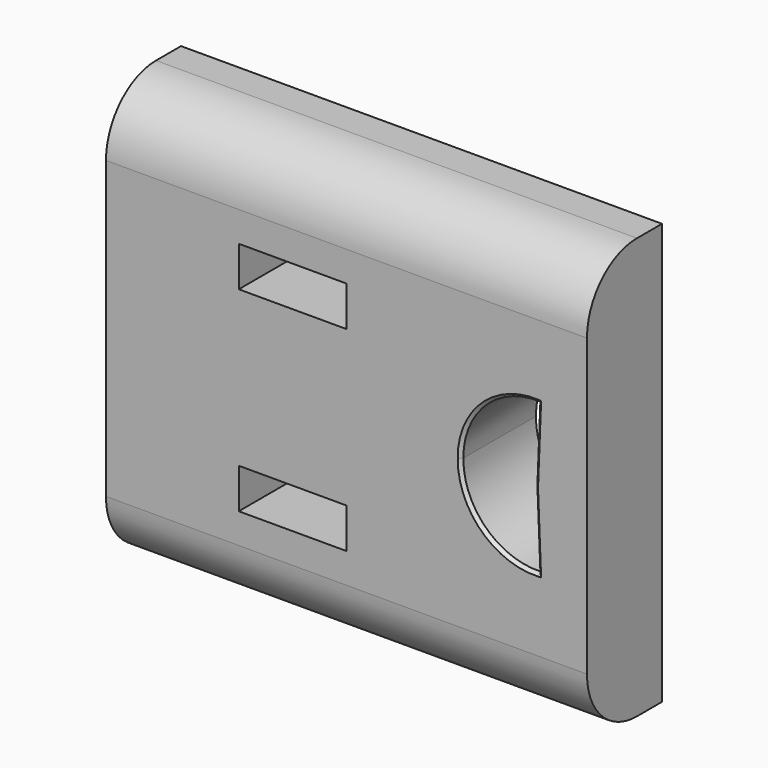
from build123d import *

# Parameters (mm, degrees)
F0_W         = 39.0713959932
F0_H         = 34.1874808073
F0_W_2       = 8.7503567338
F0_H_2       = 3.2559484243
F1_DEPTH     = 7.62
F2_R         = 5.08
F3_R         = 5.08
F4_T2_ANGLE  = 99.0884829953
F4_T4_ANGLE  = 99.0884829953
F4_T8_DEPTH  = 7.3218336241
F4_S9_R      = 6.0154186662
F4_T10_DEPTH = 5
F4_T14_DEPTH = 7.3218336241
F4_S15_R     = 6.0154186662
F4_T16_DEPTH = 5
F4_T21_DEPTH = 7.3218336241
F4_S22_R     = 6.0154186662
F4_T23_DEPTH = 5
F4_T26_ANGLE = 105.3128275547
F4_T33_ANGLE = 105.3128275547
F4_T37_DEPTH = 7.3218336241
F4_S38_R     = 6.0154186662
F4_T39_DEPTH = 5


# Not quite as in the source:
# - a fillet or chamfer that OpenCascade refuses, or shapes differently, is made with other operations: its cross-section is extruded or revolved along the edge and cut away or added


with BuildPart() as f1:
    # F0 (on Front) → F1 (new body)
    with BuildSketch(Plane.XZ):
        with Locations((19.5356979966, 17.0937404037)):
            Rectangle(F0_W, F0_H)
        with Locations((15.1605196297, 9.1573596001)):
            Rectangle(F0_W_2, F0_H_2, mode=Mode.SUBTRACT)
        with Locations((15.1605196297, 25.0301212072)):
            Rectangle(F0_W_2, F0_H_2, mode=Mode.SUBTRACT)
        with BuildLine():
            ThreePointArc((28.8283239088, 17.0937404037), (30.6523842077, 21.4714728973), (35.0814722478, 23.1670308858))
            Line((35.0814722478, 23.1670308858), (34.8434170056, 17.1563244854))
            Line((34.8434170056, 17.1563244854), (34.8434170056, 17.0311563219))
            Line((34.8434170056, 17.0311563219), (35.0814722478, 11.0204499215))
            ThreePointArc((35.0814722478, 11.0204499215), (30.6523842077, 12.71600791), (28.8283239088, 17.0937404037))
        make_face(mode=Mode.SUBTRACT)
    extrude(amount=F1_DEPTH)

    # F2
    f2_edges = [f1.edges().sort_by_distance(p)[0] for p in [
        (19.535698, -7.62, 34.187481),
    ]]
    fillet(f2_edges, radius=F2_R)

    # F3
    f3_edges = [f1.edges().sort_by_distance(p)[0] for p in [
        (19.535698, -7.62, 0),
    ]]
    fillet(f3_edges, radius=F3_R)

    # F4: chamfer of 0.254 on 4 edges, made by hand

    # F4_s1 → F4_t2 (revolve, cut)
    with BuildSketch(Plane(origin=(35.4623142005, 0, 1.4044921235), x_dir=(0, 1, 0), z_dir=(0.9992166354, 0, 0.0395741769))):
        Polygon((-7.62, 9.3694965041), (-7.366, 9.6234965041), (-7.62, 9.6234965041), align=None)
    revolve(axis=Axis((34.8434170056, -7.62, 17.0311563219), (0, 1, 0)), revolution_arc=F4_T2_ANGLE, mode=Mode.SUBTRACT)

    # F4_s3 → F4_t4 (revolve, cut)
    with BuildSketch(Plane(origin=(-1.5316236266, 0, 12.8056905764), x_dir=(0, 1, 0), z_dir=(0.1187584985, 0, -0.9929231688))):
        Polygon((-7.62, 30.3648766921), (-7.366, 30.6188766921), (-7.62, 30.6188766921), align=None)
    revolve(axis=Axis((34.8434170056, -7.62, 17.1563244854), (0, 1, 0)), revolution_arc=F4_T4_ANGLE, mode=Mode.SUBTRACT)


with BuildPart() as f4_tool6:
    # F4_s7 → F4_t8 (new body)
    with BuildSketch(Plane(origin=(0.9968897612, 0, 25.170677246), x_dir=(0, 1, 0), z_dir=(-0.0395741769, 0, -0.9992166354))):
        Polygon((-7.62, 34.3911744878), (-7.366, 34.1371744878), (-7.62, 34.1371744878), align=None)
    extrude(amount=F4_T8_DEPTH)

    # F4_s9 → F4_t10 (intersect, symmetric)
    with BuildSketch(Plane.XZ.offset(7.5)):
        with Locations((34.8434170056, 17.1563244854)):
            Circle(F4_S9_R)
    extrude(amount=F4_T10_DEPTH, both=True, mode=Mode.INTERSECT)


with BuildPart() as f1_1:
    add(f1.part)

    # F4_t5: cut F4_tool6
    add(f4_tool6.part, mode=Mode.SUBTRACT)


with BuildPart() as f4_tool12:
    # F4_s13 → F4_t14 (new body)
    with BuildSketch(Plane(origin=(-0.6447473432, 0, 16.2793599777), x_dir=(0, 1, 0), z_dir=(0.0395741769, 0, -0.9992166354))):
        Polygon((-7.62, 35.7441158998), (-7.366, 35.4901158998), (-7.62, 35.4901158998), align=None)
    extrude(amount=F4_T14_DEPTH)

    # F4_s15 → F4_t16 (intersect, symmetric)
    with BuildSketch(Plane.XZ.offset(7.5)):
        with Locations((34.8434170056, 17.0311563219)):
            Circle(F4_S15_R)
    extrude(amount=F4_T16_DEPTH, both=True, mode=Mode.INTERSECT)


with BuildPart() as f1_2:
    add(f1_1.part)

    # F4_t11: cut F4_tool12
    add(f4_tool12.part, mode=Mode.SUBTRACT)


with BuildPart() as f4_tool19:
    # F4_s20 → F4_t21 (new body)
    with BuildSketch(Plane(origin=(-0.6447473432, 0, 16.2793599777), x_dir=(0, 1, 0), z_dir=(0.0395741769, 0, -0.9992166354))):
        Polygon((-7.62, 35.7441158998), (-7.366, 35.4901158998), (-7.62, 35.4901158998), align=None)
    extrude(amount=F4_T21_DEPTH)

    # F4_s22 → F4_t23 (cut, symmetric)
    with BuildSketch(Plane.XZ.offset(7.5)):
        with Locations((34.8434170056, 17.0311563219)):
            Circle(F4_S22_R)
    extrude(amount=F4_T23_DEPTH, both=True, mode=Mode.SUBTRACT)


with BuildPart() as f4_tool24:
    # F4_s25 → F4_t26 (revolve)
    with BuildSketch(Plane(origin=(36.5710723448, 0, 5.4606046716), x_dir=(0, 1, 0), z_dir=(0.9890355378, 0, 0.1476777062))):
        Polygon((-7.62, 5.4294042858), (-7.366, 5.6834042858), (-7.62, 5.6834042858), align=None)
    revolve(axis=Axis((34.8434170056, -7.62, 17.0311563219), (0, 1, 0)), revolution_arc=F4_T26_ANGLE)

    split(bisect_by=Plane(origin=(35.4623142005, 0, 1.4044921235), x_dir=(0, 1, 0), z_dir=(0.9992166354, 0, 0.0395741769)), keep=Keep.TOP)


with BuildPart() as f4_tool19_1:
    add(f4_tool19.part)

    # F4_t28: intersect F4_tool24
    add(f4_tool24.part, mode=Mode.INTERSECT)


with BuildPart() as f1_3:
    add(f1_2.part)

    # F4_t17: cut F4_tool19
    add(f4_tool19_1.part, mode=Mode.SUBTRACT)


with BuildPart() as f4_tool31:
    # F4_s32 → F4_t33 (revolve)
    with BuildSketch(Plane(origin=(-1.5316236266, 0, 12.8056905764), x_dir=(0, 1, 0), z_dir=(0.1187584985, 0, -0.9929231688))):
        Polygon((-7.62, 30.3648766921), (-7.366, 30.6188766921), (-7.62, 30.6188766921), align=None)
    revolve(axis=Axis((34.8434170056, -7.62, 17.1563244854), (0, 1, 0)), revolution_arc=F4_T33_ANGLE)

    split(bisect_by=Plane(origin=(34.1104326349, 0, -1.3509505808), x_dir=(0, 1, 0), z_dir=(0.9992166354, 0, -0.0395741769)), keep=Keep.TOP)


with BuildPart() as f4_tool35:
    # F4_s36 → F4_t37 (new body)
    with BuildSketch(Plane(origin=(0.9968897612, 0, 25.170677246), x_dir=(0, 1, 0), z_dir=(-0.0395741769, 0, -0.9992166354))):
        Polygon((-7.62, 34.3911744878), (-7.366, 34.1371744878), (-7.62, 34.1371744878), align=None)
    extrude(amount=F4_T37_DEPTH)

    # F4_s38 → F4_t39 (cut, symmetric)
    with BuildSketch(Plane.XZ.offset(7.5)):
        with Locations((34.8434170056, 17.1563244854)):
            Circle(F4_S38_R)
    extrude(amount=F4_T39_DEPTH, both=True, mode=Mode.SUBTRACT)


with BuildPart() as f4_tool31_1:
    add(f4_tool31.part)

    # F4_t40: intersect F4_tool35
    add(f4_tool35.part, mode=Mode.INTERSECT)


with BuildPart() as f1_4:
    add(f1_3.part)

    # F4_t29: cut F4_tool31
    add(f4_tool31_1.part, mode=Mode.SUBTRACT)


solid = f1_4.part
